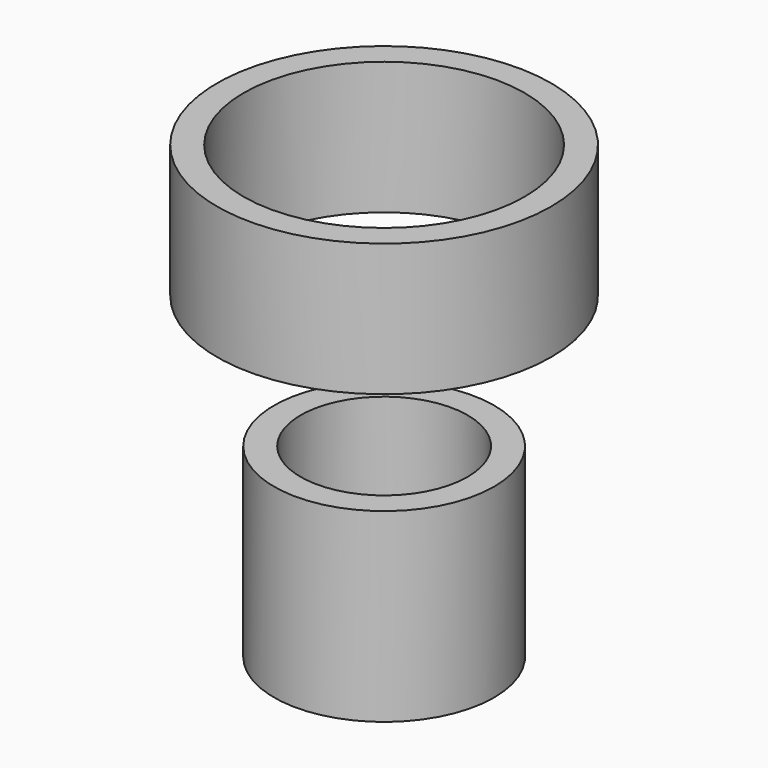
from build123d import *

# Parameters (mm, degrees)
F0_R     = 20.75
F0_R_2   = 15.75
F3_DEPTH = 35
F2_R     = 31.5
F2_R_2   = 26.5
F4_DEPTH = 25


# Not quite as in the source:
# - the program builds the solid bodies; features that only make, move or delete a surface that nothing else refers to are left out


with BuildPart() as f3:
    # F0 (on Top) → F3 (new body)
    with BuildSketch(Plane.XY):
        Circle(F0_R)
        Circle(F0_R_2, mode=Mode.SUBTRACT)
    extrude(amount=-F3_DEPTH)


with BuildPart() as f4:
    # F2 (on offset) → F4 (new body)
    with BuildSketch(Plane.XY.offset(25)):
        Circle(F2_R)
        Circle(F2_R_2, mode=Mode.SUBTRACT)
    extrude(amount=F4_DEPTH)


solid = Compound([f3.part, f4.part])
